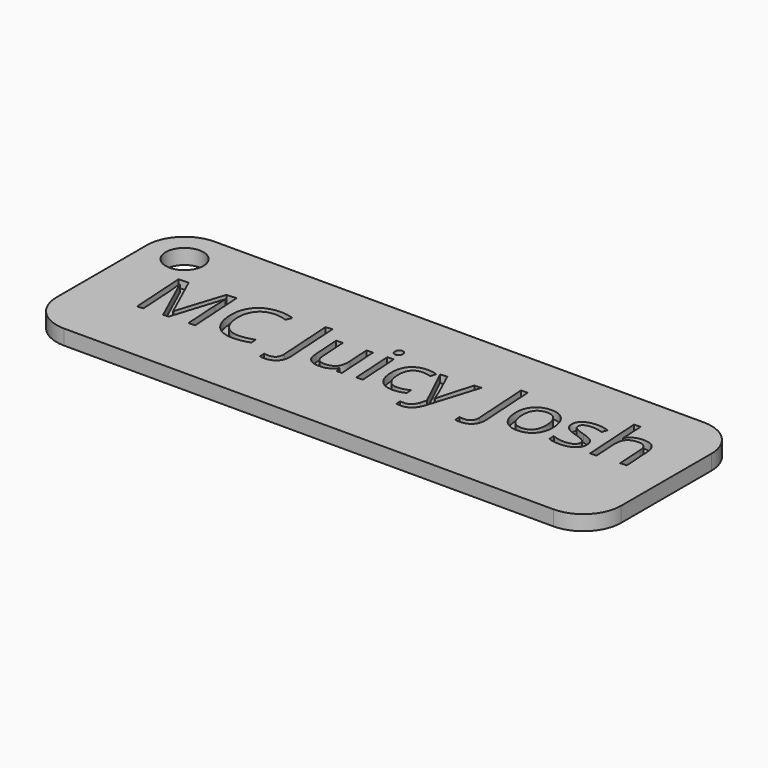
from build123d import *

# Parameters (mm, degrees)
F1_DEPTH     = 2
F3_D         = 5
F4_TEXT_SIZE = 10.4366905468
F5_DEPTH     = 1


# Not quite as in the source:
# - Text() gives the source's letters only with a copy of the font that has no kerning and outlines rounded to 1/6400 em; it was checked with that copy


with BuildPart() as f1:
    # F0 (on Top) → F1 (new body)
    with BuildSketch(Plane.XY):
        with BuildLine():
            Line((32.5, 12.5), (-32.5, 12.5))
            ThreePointArc((-32.5, 12.5), (-36.0355339059, 11.0355339059), (-37.5, 7.5))
            Line((-37.5, 7.5), (-37.5, -7.5))
            ThreePointArc((-37.5, -7.5), (-36.0355339059, -11.0355339059), (-32.5, -12.5))
            Line((-32.5, -12.5), (32.5, -12.5))
            ThreePointArc((32.5, -12.5), (36.0355339059, -11.0355339059), (37.5, -7.5))
            Line((37.5, -7.5), (37.5, 7.5))
            ThreePointArc((37.5, 7.5), (36.0355339059, 11.0355339059), (32.5, 12.5))
        make_face()
    extrude(amount=F1_DEPTH)

    # F3 (through all)
    with Locations(Plane.XY.offset(2)):
        with Locations((-32.5, 7.5)):
            Hole(F3_D / 2)

    # F4 (on face) → F5 (cut)
    with BuildSketch(Plane.XY.offset(2)):
        with Locations(Location((-30.7163818138, -3.9504592554), (0, 0, 3.5497666666))):
            Text('MC Juicy Josh', F4_TEXT_SIZE, font='Open Sans', text_align=(TextAlign.LEFT, TextAlign.BOTTOM))
    extrude(amount=-F5_DEPTH, mode=Mode.SUBTRACT)


solid = f1.part
